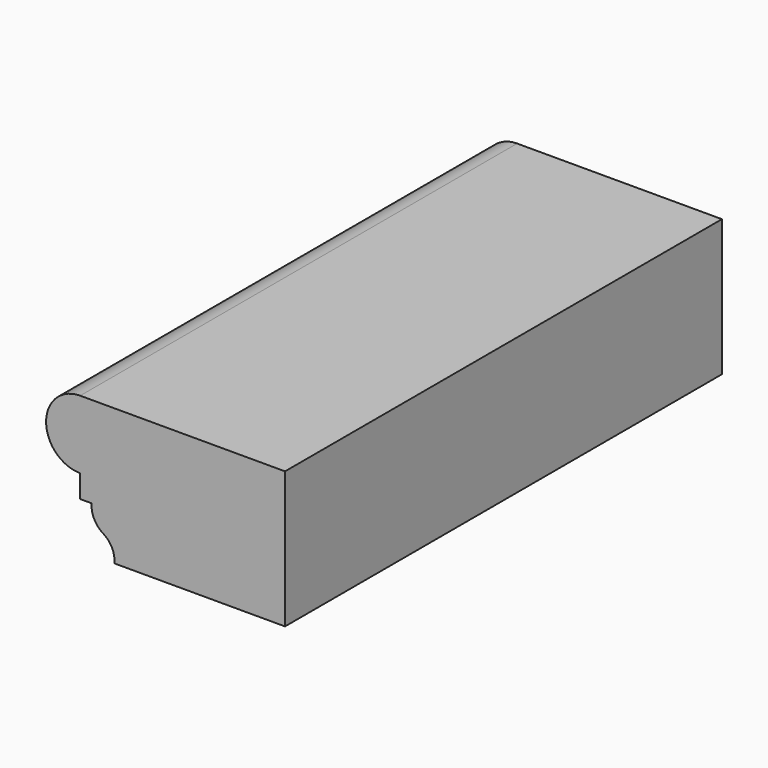
from build123d import *

# Parameters (mm, degrees)
F0_W     = 38.1
F0_H     = 19.05
F0_H_2   = 19.0520574
F1_DEPTH = 152.4


# Not quite as in the source:
# - ends of sketch curves that miss each other by under 0.0002 mm in the source are joined


with BuildPart() as f1:
    # F0 (on Front) → F1 (new body)
    with BuildSketch(Plane.XZ):
        with Locations((14.288262, -9.5260414)):
            Rectangle(F0_W, F0_H)
        with BuildLine():
            Line((-14.287246, -19.0510414), (-4.761738, -19.0510414))
            Line((-4.761738, -19.0510414), (-4.761738, -0.0010414))
            Line((-4.761738, -0.0010414), (-4.761738, 19.051016))
            Line((-4.761738, 19.051016), (-23.812754, 19.051016))
            ThreePointArc((-23.812754, 19.051016), (-30.548305301, 16.261059301), (-33.338262, 9.525508))
            ThreePointArc((-33.338262, 9.525508), (-30.548305301, 2.789956699), (-23.812754, 0))
            Line((-23.812754, 0), (-23.812754, -6.3503556))
            Line((-23.812754, -6.3503556), (-20.6375762, -6.3503556))
            ThreePointArc((-20.6375762, -6.3503556), (-19.9375622279, -9.969300362), (-17.4624299923, -12.700695633))
            ThreePointArc((-17.4624299923, -12.700695633), (-14.947472994, -15.4121856415), (-14.287246, -19.0510414))
        make_face()
        with Locations((14.288262, 9.5249873)):
            Rectangle(F0_W, F0_H_2)
    extrude(amount=F1_DEPTH)


solid = f1.part
